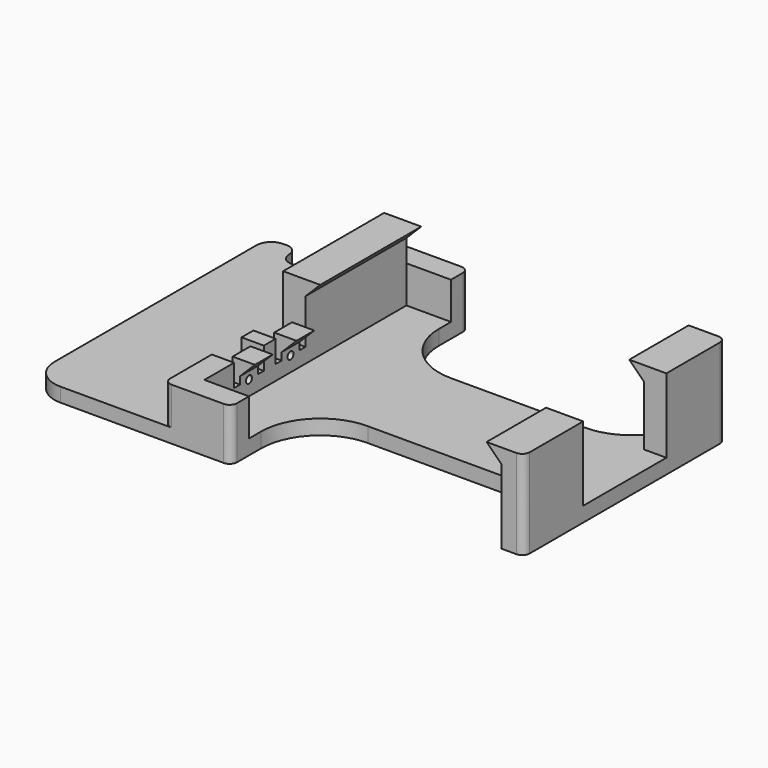
from build123d import *

# Parameters (mm, degrees)
F1_DEPTH  = 2
F2_W      = 3
F2_H      = 17
F3_DEPTH  = 10
F4_W      = 10
F4_H      = 2
F5_DEPTH  = 2
F6_SIZE   = 1.99999
F2_H_2    = 10
F2_H_3    = 7
F7_DEPTH  = 5
F8_DEPTH  = 7
F9_W      = 17
F9_H      = 2
F10_DEPTH = 2
F11_SIZE  = 1.99999
F14_DEPTH = 2
F15_SIZE  = 1.99999
F17_DEPTH = 3
F18_R     = 0.5
F19_DEPTH = 3.001
F21_DEPTH = 1.9


# Not quite as in the source:
# - a fillet or chamfer is up to 0.001 mm smaller than in the source, because OpenCascade refuses the exact size
# - a feature names something its author has since deleted; it is built from what else it names


with BuildPart() as f1:
    # F0 (on Top) → F1 (new body)
    with BuildSketch(Plane.XY):
        with BuildLine():
            Line((-14, 17), (-15, 17))
            Line((-15, 17), (-20, 17))
            Line((-20, 17), (-20, -15))
            Line((-20, -15), (-20, -17))
            Line((-20, -17), (-15, -17))
            Line((-15, -17), (-14, -17))
            Line((-14, -17), (-14, -15))
            ThreePointArc((-14, -15), (-11.6568542495, -9.3431457505), (-6, -7))
            Line((-6, -7), (12, -7))
            ThreePointArc((12, -7), (17.6568542495, -9.3431457505), (20, -15))
            Line((20, -15), (20, 15))
            ThreePointArc((20, 15), (17.6568542495, 9.3431457505), (12, 7))
            Line((12, 7), (-6, 7))
            ThreePointArc((-6, 7), (-11.6568542495, 9.3431457505), (-14, 15))
            Line((-14, 15), (-14, 17))
        make_face()
        Polygon((-20, -15), (-20, 17), (-23, 17), (-23, -17), (-20, -17), align=None)
        with BuildLine():
            Line((22, 17), (20, 17))
            Line((20, 17), (20, 15))
            Line((20, 15), (20, -15))
            Line((20, -15), (20, -17))
            Line((20, -17), (22, -17))
            ThreePointArc((22, -17), (22.7071067812, -16.7071067812), (23, -16))
            Line((23, -16), (23, 16))
            ThreePointArc((23, 16), (22.7071067812, 16.7071067812), (22, 17))
        make_face()
    extrude(amount=F1_DEPTH)

    # F2 (on face) → F3 (join)
    with BuildSketch(Plane.XY.offset(2)):
        with BuildLine():
            Line((20, -7), (20, -15))
            Line((20, -15), (20, -17))
            Line((20, -17), (22, -17))
            ThreePointArc((22, -17), (22.7071067812, -16.7071067812), (23, -16))
            Line((23, -16), (23, -7))
            Line((23, -7), (20, -7))
        make_face()
        with BuildLine():
            Line((20, 15), (20, 7))
            Line((20, 7), (23, 7))
            Line((23, 7), (23, 16))
            ThreePointArc((23, 16), (22.7071067812, 16.7071067812), (22, 17))
            Line((22, 17), (20, 17))
            Line((20, 17), (20, 15))
        make_face()
        with Locations((-21.5, 8.5)):
            Rectangle(F2_W, F2_H)
    extrude(amount=F3_DEPTH)

    # F4 (on face) → F5 (join)
    with BuildSketch(Plane(origin=(20, 0, 0), x_dir=(0, -1, 0), z_dir=(-1, 0, 0))):
        with Locations((-12, 11)):
            Rectangle(F4_W, F4_H)
        with Locations((12, 11)):
            Rectangle(F4_W, F4_H)
    extrude(amount=F5_DEPTH)

    # F6 (size 2 in the source; OpenCascade refuses exactly that, so slightly less here)
    f6_edges = [f1.edges().sort_by_distance(p)[0] for p in [
        (18, 12, 10),
        (18, -12, 10),
    ]]
    chamfer(f6_edges, length=F6_SIZE)

    # F2 (on face) → F7 (join)
    with BuildSketch(Plane.XY.offset(2)):
        with Locations((-21.5, -12)):
            Rectangle(F2_W, F2_H_2)
        with Locations((-21.5, -3.5)):
            Rectangle(F2_W, F2_H_3)
    extrude(amount=F7_DEPTH)

    # F0 (on Top) → F8 (join)
    with BuildSketch(Plane.XY):
        with BuildLine():
            Line((-15, -17), (-20, -17))
            Line((-20, -17), (-23, -17))
            Line((-23, -17), (-23, -19))
            ThreePointArc((-23, -19), (-22.7071067812, -19.7071067812), (-22, -20))
            Line((-22, -20), (-15, -20))
            ThreePointArc((-15, -20), (-14.2928932188, -19.7071067812), (-14, -19))
            Line((-14, -19), (-14, -18))
            Line((-14, -18), (-14, -17))
            Line((-14, -17), (-15, -17))
        make_face()
        with BuildLine():
            Line((-20, 17), (-15, 17))
            Line((-15, 17), (-14, 17))
            Line((-14, 17), (-14, 18))
            Line((-14, 18), (-14, 19))
            ThreePointArc((-14, 19), (-14.2928932188, 19.7071067812), (-15, 20))
            Line((-15, 20), (-22, 20))
            ThreePointArc((-22, 20), (-22.7071067812, 19.7071067812), (-23, 19))
            Line((-23, 19), (-23, 17))
            Line((-23, 17), (-20, 17))
        make_face()
    extrude(amount=F8_DEPTH)

    # F9 (on face) → F10 (join)
    with BuildSketch(Plane.YZ.offset(-20)):
        with Locations((8.5, 11)):
            Rectangle(F9_W, F9_H)
    extrude(amount=F10_DEPTH)

    # F11 (size 2 in the source; OpenCascade refuses exactly that, so slightly less here)
    f11_edges = [f1.edges().sort_by_distance(p)[0] for p in [
        (-18, 8.5, 10),
    ]]
    chamfer(f11_edges, length=F11_SIZE)

    # F13 (on face) → F14 (join)
    with BuildSketch(Plane.YZ.offset(-20)):
        Polygon((-9.5, 7), (-11, 7), (-11, 5), (-8, 5), (-8, 7), align=None)
        Polygon((-1, 5), (-1, 7), (-2.5, 7), (-4, 7), (-4, 5), align=None)
    extrude(amount=F14_DEPTH)

    # F15 (size 2 in the source; OpenCascade refuses exactly that, so slightly less here)
    f15_edges = [f1.edges().sort_by_distance(p)[0] for p in [
        (-18, -9.5, 5),
        (-18, -2.5, 5),
    ]]
    chamfer(f15_edges, length=F15_SIZE)

    # F16 (on face) → F17 (cut)
    with BuildSketch(Plane.XY.offset(7)):
        Polygon((-23, 0), (-23, -1), (-23, -4), (-21, -4), (-21, -1), (-20, -1), (-20, 0), align=None)
        Polygon((-21, -4), (-23, -4), (-23, -5), (-20, -5), (-20, -4), align=None)
        Polygon((-21, -8), (-23, -8), (-23, -11), (-23, -12), (-21, -12), (-20, -12), (-20, -11), (-21, -11), align=None)
        Polygon((-21, -7), (-23, -7), (-23, -8), (-21, -8), (-20, -8), (-20, -7), align=None)
    extrude(amount=-F17_DEPTH, mode=Mode.SUBTRACT)

    # F18 (on face) → F19 (cut, through all)
    with BuildSketch(Plane.YZ.offset(-20)):
        with Locations((-9.5, 4)):
            Circle(F18_R)
        with Locations((-2.5, 4)):
            Circle(F18_R)
    extrude(amount=-F19_DEPTH, mode=Mode.SUBTRACT)

    # F20 (on Top) → F21 (join)
    with BuildSketch(Plane.XY):
        with BuildLine():
            Line((-23, -19), (-23, -17))
            Line((-23, -17), (-23, 17))
            Line((-23, 17), (-23, 19))
            Line((-23, 19), (-23, 20))
            Line((-23, 20), (-25.5, 20))
            ThreePointArc((-25.5, 20), (-26.5606601718, 19.5606601718), (-27, 18.5))
            ThreePointArc((-27, 18.5), (-27.4393398282, 17.4393398282), (-28.5, 17))
            Line((-28.5, 17), (-35.5, 17))
            ThreePointArc((-35.5, 17), (-36.5606601718, 17.4393398282), (-37, 18.5))
            ThreePointArc((-37, 18.5), (-37.4393398282, 19.5606601718), (-38.5, 20))
            Line((-38.5, 20), (-39, 20))
            ThreePointArc((-39, 20), (-40.4142135624, 19.4142135624), (-41, 18))
            Line((-41, 18), (-41, 16))
            Line((-41, 16), (-41, -16))
            ThreePointArc((-41, -16), (-39.8284271247, -18.8284271247), (-37, -20))
            Line((-37, -20), (-23, -20))
            Line((-23, -20), (-23, -19))
        make_face()
        with BuildLine():
            Line((-23, 20), (-23, 19))
            ThreePointArc((-23, 19), (-22.7071067812, 19.7071067812), (-22, 20))
            Line((-22, 20), (-23, 20))
        make_face()
        with BuildLine():
            ThreePointArc((-22, -20), (-22.7071067812, -19.7071067812), (-23, -19))
            Line((-23, -19), (-23, -20))
            Line((-23, -20), (-22, -20))
        make_face()
    extrude(amount=F21_DEPTH)


solid = f1.part
